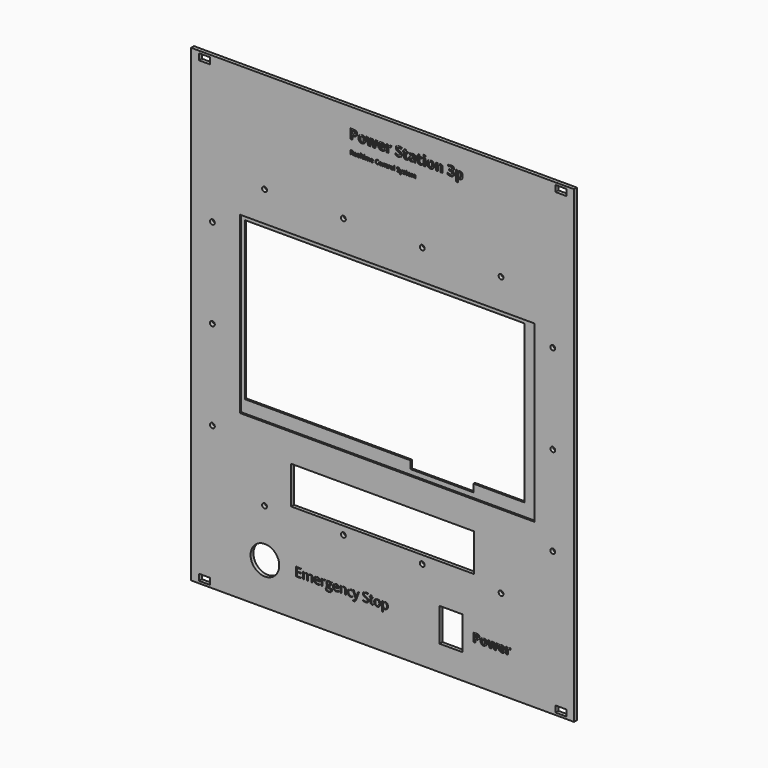
from build123d import *

# Parameters (mm, degrees)
F0_W            = 213.75
F0_H            = 261.75
F1_DEPTH        = 2
F2_R            = 8
F3_DEPTH        = 25
F4_W            = 13
F4_H            = 18.6
F5_DEPTH        = 25
F6_TEXT_SIZE    = 6.9330896856
F7_DEPTH        = 0.5
F8_TEXT_SIZE    = 6.7874158039
F9_DEPTH        = 0.5
F10_R           = 1.35
F11_DEPTH       = 25
F12_W           = 102
F12_H           = 21
F13_DEPTH       = 25
F14_W           = 156
F14_H           = 88
F15_DEPTH       = 25
F16_TEXT_SIZE   = 7.5057976776
F16_TEXT_SIZE_2 = 3.2167674767
F17_DEPTH       = 0.5
F18_W           = 6.1
F18_H           = 3.5
F19_DEPTH       = 25
F20_W           = 164.5
F20_H           = 97.5
F21_DEPTH       = 1
F22_W           = 35
F22_H           = 11.1636901496
F23_DEPTH       = 25


# Not quite as in the source:
# - Text() gives the source's letters only with a copy of the font that has no kerning and outlines rounded to 1/6400 em; it was checked with that copy


with BuildPart() as f1:
    # F0 (on Front) → F1 (new body)
    with BuildSketch(Plane.XZ):
        with Locations((106.875, 130.875)):
            Rectangle(F0_W, F0_H)
    extrude(amount=-F1_DEPTH)

    # F2 (on Front) → F3 (cut)
    with BuildSketch(Plane.XZ):
        with Locations((41.21, 23.32)):
            Circle(F2_R)
    extrude(amount=-F3_DEPTH, mode=Mode.SUBTRACT)

    # F4 (on face) → F5 (cut)
    with BuildSketch(Plane.XZ):
        with Locations((145.1, 23.32)):
            Rectangle(F4_W, F4_H)
    extrude(amount=-F5_DEPTH, mode=Mode.SUBTRACT)

    # F6 (on face) → F7 (cut)
    with BuildSketch(Plane.XZ):
        with Locations((58, 21)):
            Text('Emergency Stop', F6_TEXT_SIZE, font='Open Sans', text_align=(TextAlign.LEFT, TextAlign.BOTTOM))
    extrude(amount=-F7_DEPTH, mode=Mode.SUBTRACT)

    # F8 (on face) → F9 (cut)
    with BuildSketch(Plane.XZ):
        with Locations((157, 21)):
            Text('Power', F8_TEXT_SIZE, font='Open Sans', font_style=FontStyle.BOLD, text_align=(TextAlign.LEFT, TextAlign.BOTTOM))
    extrude(amount=-F9_DEPTH, mode=Mode.SUBTRACT)

    # F10 (on face) → F11 (cut)
    with BuildSketch(Plane.XZ):
        with Locations((41, 50)):
            Circle(F10_R)
        with Locations((85, 50)):
            Circle(F10_R)
        with Locations((129, 50)):
            Circle(F10_R)
        with Locations((173, 50)):
            Circle(F10_R)
        with Locations((41, 205.5)):
            Circle(F10_R)
        with Locations((85, 205.5)):
            Circle(F10_R)
        with Locations((129, 205.5)):
            Circle(F10_R)
        with Locations((173, 205.5)):
            Circle(F10_R)
        with Locations((11.88, 80)):
            Circle(F10_R)
        with Locations((201.88, 80)):
            Circle(F10_R)
        with Locations((201.88, 130)):
            Circle(F10_R)
        with Locations((11.88, 130)):
            Circle(F10_R)
        with Locations((11.88, 180)):
            Circle(F10_R)
        with Locations((201.88, 180)):
            Circle(F10_R)
    extrude(amount=-F11_DEPTH, mode=Mode.SUBTRACT)

    # F12 (on face) → F13 (cut)
    with BuildSketch(Plane.XZ):
        with Locations((106.88, 65)):
            Rectangle(F12_W, F12_H)
    extrude(amount=-F13_DEPTH, mode=Mode.SUBTRACT)

    # F14 (on face) → F15 (cut)
    with BuildSketch(Plane.XZ):
        with Locations((107.16, 142.15)):
            Rectangle(F14_W, F14_H)
    extrude(amount=-F15_DEPTH, mode=Mode.SUBTRACT)

    # F16 (on face) → F17 (cut)
    with BuildSketch(Plane.XZ):
        with Locations((88.2896184921, 245.8499670029)):
            Text('Power Station 3p', F16_TEXT_SIZE, font='Open Sans', font_style=FontStyle.BOLD, text_align=(TextAlign.LEFT, TextAlign.BOTTOM))
        with Locations((88.6756330729, 238.2621765137)):
            Text('Realtime Control System', F16_TEXT_SIZE_2, font='Open Sans', text_align=(TextAlign.LEFT, TextAlign.BOTTOM))
    extrude(amount=-F17_DEPTH, mode=Mode.SUBTRACT)

    # F18 (on face) → F19 (cut)
    with BuildSketch(Plane.XZ):
        with Locations((7.45, 3)):
            Rectangle(F18_W, F18_H)
        with Locations((206.45, 3)):
            Rectangle(F18_W, F18_H)
        with Locations((206.45, 258.75)):
            Rectangle(F18_W, F18_H)
        with Locations((7.45, 258.75)):
            Rectangle(F18_W, F18_H)
    extrude(amount=-F19_DEPTH, mode=Mode.SUBTRACT)

    # F20 (on face) → F21 (cut)
    with BuildSketch(Plane.XZ):
        with Locations((109.45, 139.87)):
            Rectangle(F20_W, F20_H)
    extrude(amount=-F21_DEPTH, mode=Mode.SUBTRACT)

    # F22 (on face) → F23 (cut)
    with BuildSketch(Plane.XZ.offset(-1)):
        with Locations((139.2, 99.4364432991)):
            Rectangle(F22_W, F22_H)
    extrude(amount=-F23_DEPTH, mode=Mode.SUBTRACT)


solid = f1.part
